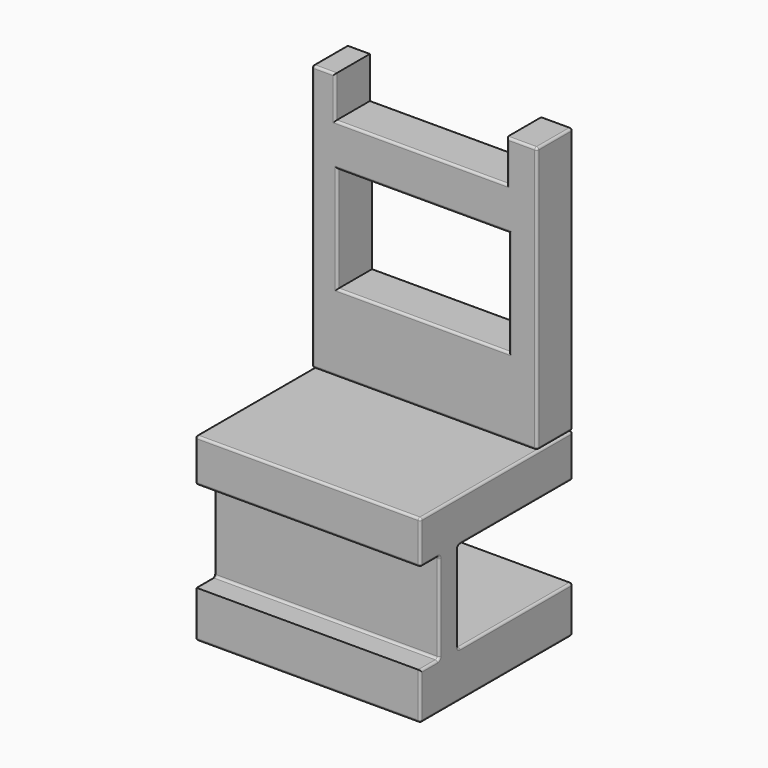
from build123d import *

# Parameters (mm, degrees)
F0_W     = 9.9436193705
F0_H     = 59.1063983738
F1_DEPTH = 50
F0_W_2   = 5.2507026121
F0_H_2   = 20.0943984091
F2_W     = 38.0825251341
F2_H     = 23.3743079007
F2_W_2   = 38.0357308313
F2_H_2   = 12.3214237392
F3_DEPTH = 25
F4_R     = 0.5
F4_2_R   = 0.5


with BuildPart() as f1:
    # F0 (on Right) → F1 (new body)
    with BuildSketch(Plane.YZ):
        with Locations((-4.9718096852, 39.2434578389)):
            Rectangle(F0_W, F0_H)
    extrude(amount=F1_DEPTH)

    # F2 (on Front) → F3 (cut)
    with BuildSketch(Plane.XZ):
        with Locations((24.7360542417, 38.5746154934)):
            Rectangle(F2_W, F2_H)
        with Locations((24.241077248, 65.7589305192)):
            Rectangle(F2_W_2, F2_H_2)
    extrude(amount=F3_DEPTH, mode=Mode.SUBTRACT)

    # F4
    f4_edges = [f1.edges().sort_by_distance(p)[0] for p in [
        (0, -9.943619, 39.243458),
        (25, -9.943619, 9.690259),
        (50, -9.943619, 39.243458),
        (46.629471, -9.943619, 68.796657),
        (43.258943, -9.943619, 64.197438),
        (24.241077, -9.943619, 59.598219),
        (5.223212, -9.943619, 64.197438),
        (2.611606, -9.943619, 68.796657),
        (24.736054, -9.943619, 50.261769),
        (43.777317, -9.943619, 38.574615),
        (24.736054, -9.943619, 26.887462),
        (5.694792, -9.943619, 38.574615),
        (0, 0, 39.243458),
        (0, -4.97181, 68.796657),
        (0, -4.97181, 9.690259),
        (50, 0, 39.243458),
        (50, -4.97181, 68.796657),
        (50, -4.97181, 9.690259),
        (2.611606, 0, 68.796657),
        (5.223212, 0, 64.197438),
        (24.241077, 0, 59.598219),
        (43.258943, 0, 64.197438),
        (46.629471, 0, 68.796657),
        (25, 0, 9.690259),
        (5.694792, 0, 38.574615),
        (24.736054, 0, 26.887462),
        (43.777317, 0, 38.574615),
        (24.736054, 0, 50.261769),
    ]]
    fillet(f4_edges, radius=F4_R)


with BuildPart() as f1b:
    # F0 (on Right) → F1, piece 2 (new body)
    with BuildSketch(Plane.YZ):
        Polygon((-31.7991506308, 0), (0, 0), (0, 9.5437960699), (-42.300555855, 9.5437960699), (-42.300555855, 0), (-37.0498532429, 0), align=None)
        with Locations((-34.4245019369, -10.0471992046)):
            Rectangle(F0_W_2, F0_H_2)
        Polygon((0, -20.0943984091), (-31.7991506308, -20.0943984091), (-37.0498532429, -20.0943984091), (-42.300555855, -20.0943984091), (-42.300555855, -30.4523352534), (0, -30.4523352534), align=None)
    extrude(amount=F1_DEPTH)

    # F4#2
    f4_2_edges = [f1b.edges().sort_by_distance(p)[0] for p in [
        (25, 0, 9.543796),
        (25, -42.300556, 9.543796),
        (0, -21.150278, 9.543796),
        (50, -21.150278, 9.543796),
        (0, -15.899575, 0),
        (0, 0, 4.771898),
        (0, -42.300556, 4.771898),
        (0, -39.675205, 0),
        (0, -37.049853, -10.047199),
        (0, -39.675205, -20.094398),
        (0, -42.300556, -25.273367),
        (0, -21.150278, -30.452335),
        (0, 0, -25.273367),
        (0, -15.899575, -20.094398),
        (0, -31.799151, -10.047199),
        (25, -42.300556, 0),
        (25, -37.049853, 0),
        (25, -37.049853, -20.094398),
        (50, -37.049853, -10.047199),
        (25, -42.300556, -30.452335),
        (50, -15.899575, 0),
        (50, 0, 4.771898),
        (50, -42.300556, 4.771898),
        (50, -39.675205, 0),
        (50, -39.675205, -20.094398),
        (50, -42.300556, -25.273367),
        (50, -21.150278, -30.452335),
        (50, 0, -25.273367),
        (50, -15.899575, -20.094398),
        (50, -31.799151, -10.047199),
        (25, 0, 0),
        (25, -31.799151, -20.094398),
        (25, -31.799151, 0),
        (25, 0, -20.094398),
        (25, 0, -30.452335),
    ]]
    fillet(f4_2_edges, radius=F4_2_R)


solid = Compound([f1.part, f1b.part])
